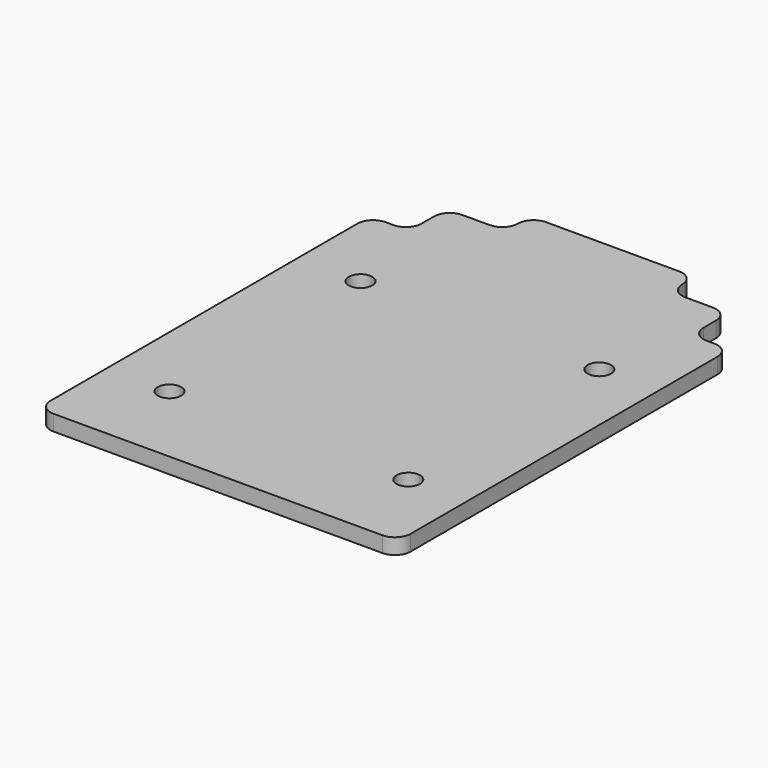
from build123d import *

# Parameters (mm, degrees)
F0_R     = 1.5
F1_DEPTH = 2
F2_R     = 1.99999


# Not quite as in the source:
# - a fillet or chamfer is up to 0.001 mm smaller than in the source, because OpenCascade refuses the exact size


with BuildPart() as f1:
    # F0 (on Top) → F1 (new body)
    with BuildSketch(Plane.XY):
        Polygon((10.5, 31.5), (-10.5, 31.5), (-10.5, 27.5), (-18, 27.5), (-18, 21.5), (-23, 21.5), (-23, -31.5), (23, -31.5), (23, 21.5), (18, 21.5), (18, 27.5), (10.5, 27.5), align=None)
        with Locations((-15, -20.5)):
            Circle(F0_R, mode=Mode.SUBTRACT)
        with Locations((15.5, -20.5)):
            Circle(F0_R, mode=Mode.SUBTRACT)
        with Locations((-15, 10)):
            Circle(F0_R, mode=Mode.SUBTRACT)
        with Locations((15.5, 10)):
            Circle(F0_R, mode=Mode.SUBTRACT)
    extrude(amount=F1_DEPTH)

    # F2 (radius 2 in the source; OpenCascade refuses exactly that, so slightly less here)
    f2_edges = [f1.edges().sort_by_distance(p)[0] for p in [
        (10.5, 31.5, 1),
        (23, 21.5, 1),
        (18, 27.5, 1),
        (18, 21.5, 1),
        (10.5, 27.5, 1),
        (-10.5, 31.5, 1),
        (-10.5, 27.5, 1),
        (-18, 27.5, 1),
        (-18, 21.5, 1),
        (-23, 21.5, 1),
        (-23, -31.5, 1),
        (23, -31.5, 1),
    ]]
    fillet(f2_edges, radius=F2_R)


solid = f1.part
